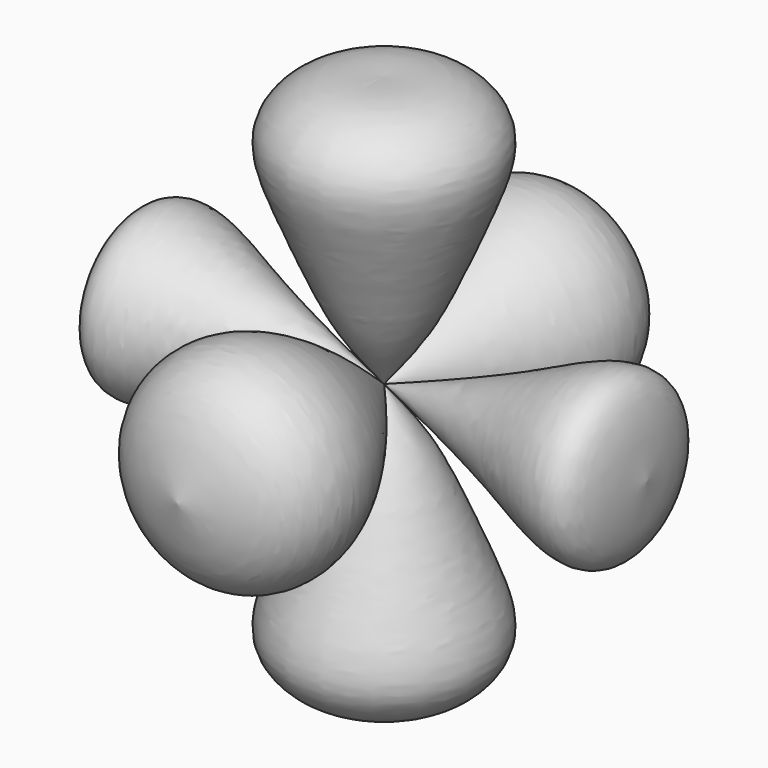
from build123d import *


# Not quite as in the source:
# - a feature names something its author has since deleted; it is built from what else it names


with BuildPart() as f1:
    # F0 (on Right) → F1 (revolve)
    with BuildSketch(Plane.YZ):
        with BuildLine():
            Line((0, 0), (0, 59.2521093786))
            add(Edge.make_bspline(
                [(0, 59.2521093786), (-4.7387822155, 59.4274798173), (-13.9165550358, 59.7671261596), (-24.7844658436, 49.6650341304), (-19.7844391022, 35.8879005927), (-13.9477352777, 22.2650438348), (-8.5895348934, 10.6607669), (-2.8953275907, 3.5934905588), (0, 0)],
                knots=[0, 0, 0, 0, 0.1688062696, 0.3269332759, 0.4924602589, 0.6700430734, 0.832227149, 1, 1, 1, 1], degree=3))
        make_face()
    revolve(axis=Axis((0, 0, 0), (0, 0, -1)))



with BuildPart() as f1b:
    # F0 (on Right) → F1, piece 2 (revolve)
    with BuildSketch(Plane.YZ):
        with BuildLine():
            Line((0, -59.2521093786), (0, 0))
            add(Edge.make_bspline(
                [(0, -59.2521093786), (-4.7387822155, -59.4274798173), (-13.9165550358, -59.7671261596), (-24.7844658436, -49.6650341304), (-19.7844391022, -35.8879005927), (-13.9477352777, -22.2650438348), (-8.5895348934, -10.6607669), (-2.8953275907, -3.5934905588), (0, 0)],
                knots=[0, 0, 0, 0, 0.1688062696, 0.3269332759, 0.4924602589, 0.6700430734, 0.832227149, 1, 1, 1, 1], degree=3))
        make_face()
    revolve(axis=Axis((0, 0, 0), (0, 0, -1)))


with BuildPart() as f1_1:
    add(f1.part)

    add(f1b.part)  # F3 merges F1b
    # F2 (on Front) → F3 (revolve)
    with BuildSketch(Plane.XZ):
        with BuildLine():
            Line((0, 0), (-57.5616061687, 0))
            add(Edge.make_bspline(
                [(0, 0), (-10.4737408609, -3.7347990618), (-29.3560288191, -10.4679760888), (-55.1891100393, -23.9292829099), (-57.1008358167, -3.4689589587), (-57.4466807158, -0.8652285848), (-57.5616061687, 0)],
                knots=[0, 0, 0, 0, 0.3593590005, 0.6478602266, 0.8829827386, 1, 1, 1, 1], degree=3))
        make_face()
        with BuildLine():
            Line((57.5616061687, 0), (0, 0))
            add(Edge.make_bspline(
                [(0, 0), (10.4737408609, -3.7347990618), (29.3560288191, -10.4679760888), (55.1891100393, -23.9292829099), (57.1008358167, -3.4689589587), (57.4466807158, -0.8652285848), (57.5616061687, 0)],
                knots=[0, 0, 0, 0, 0.3593590005, 0.6478602266, 0.8829827386, 1, 1, 1, 1], degree=3))
        make_face()
    revolve(axis=Axis((0.0845249742, 0, 0), (1, 0, 0)))


with BuildPart() as f5:
    # F4 (on Top) → F5 (revolve)
    with BuildSketch(Plane.XY):
        with BuildLine():
            add(Edge.make_bspline(
                [(0, 0), (-9.8761914078, -11.3902021624), (-26.2547427816, -30.2795698926), (-20.3828318801, -52.4204355109), (-6.9188317465, -55.2420643448), (0.0165426494, -56.6954995925)],
                knots=[0, 0, 0, 0, 0.4241252859, 0.7033640294, 1, 1, 1, 1], degree=3))
            Line((0.0165426494, -56.6954995925), (0.0165426494, 56.6954995925))
            add(Edge.make_bspline(
                [(0, 0), (-9.8761914078, 11.3902021624), (-26.2547427816, 30.2795698926), (-20.3828318801, 52.4204355109), (-6.9188317465, 55.2420643448), (0.0165426494, 56.6954995925)],
                knots=[0, 0, 0, 0, 0.4241252859, 0.7033640294, 1, 1, 1, 1], degree=3))
        make_face()
    revolve(axis=Axis((0.0165426494, 0, 0), (0, 1, 0)))


solid = Compound([f1_1.part, f5.part])
